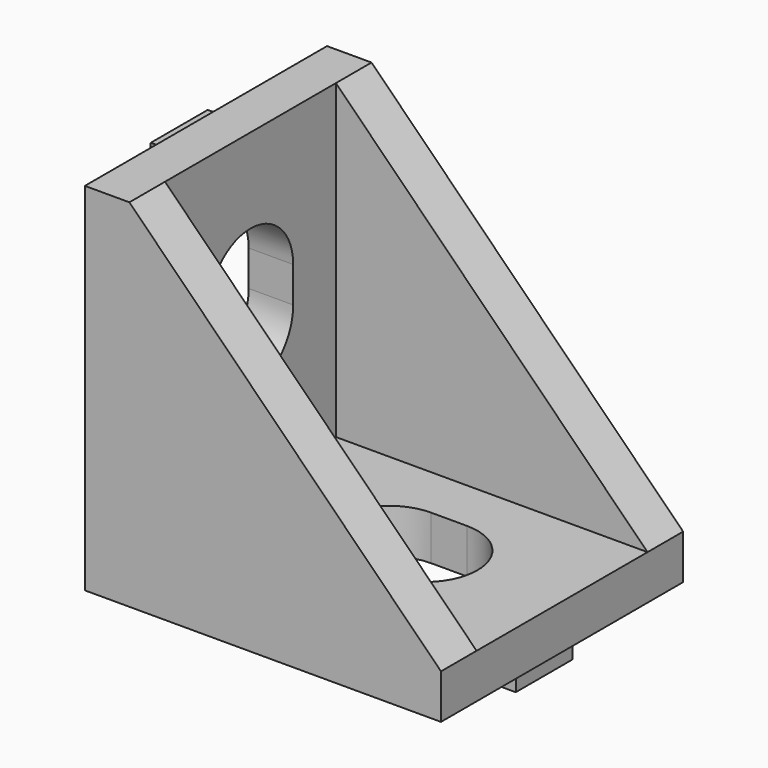
from build123d import *

# Parameters (mm, degrees)
F0_W     = 2.5
F0_H     = 8
F0_W_2   = 8
F0_H_2   = 2.5
F1_DEPTH = 17
F2_START = 2.5
F2_DEPTH = 12
F3_START = 5.5
F3_DEPTH = 6
F4_R     = 2.99999
F5_START = 6.5
F0_W_3   = 1.5
F0_H_3   = 1.5
F5_DEPTH = 4


# Not quite as in the source:
# - a fillet or chamfer is up to 0.001 mm smaller than in the source, because OpenCascade refuses the exact size


with BuildPart() as f1:
    # F0 (on Front) → F1 (new body)
    with BuildSketch(Plane.XZ):
        Polygon((20, 2.5), (2.5, 20), (2.5, 15.25), (2.5, 7.25), (2.5, 2.5), (7.25, 2.5), (15.25, 2.5), align=None)
        Polygon((20, 0), (20, 2.5), (15.25, 2.5), (15.25, 0), (16.5, 0), (19, 0), align=None)
        Polygon((2.5, 20), (0, 20), (0, 19), (0, 16.5), (0, 15.25), (2.5, 15.25), align=None)
        Polygon((2.5, 2.5), (2.5, 7.25), (0, 7.25), (0, 6), (0, 3.5), (0, 0), (3.5, 0), (6, 0), (7.25, 0), (7.25, 2.5), align=None)
        with Locations((1.25, 11.25)):
            Rectangle(F0_W, F0_H)
        with Locations((11.25, 1.25)):
            Rectangle(F0_W_2, F0_H_2)
    extrude(amount=F1_DEPTH)

    # F0 (on Front) → F2 (cut)
    with BuildSketch(Plane.XZ.offset(F2_START)):
        Polygon((20, 2.5), (2.5, 20), (2.5, 15.25), (2.5, 7.25), (2.5, 2.5), (7.25, 2.5), (15.25, 2.5), align=None)
    extrude(amount=F2_DEPTH, mode=Mode.SUBTRACT)

    # F0 (on Front) → F3 (cut)
    with BuildSketch(Plane.XZ.offset(F3_START)):
        with Locations((1.25, 11.25)):
            Rectangle(F0_W, F0_H)
        with Locations((11.25, 1.25)):
            Rectangle(F0_W_2, F0_H_2)
    extrude(amount=F3_DEPTH, mode=Mode.SUBTRACT)

    # F4 (radius 3 in the source; OpenCascade refuses exactly that, so slightly less here)
    f4_edges = [f1.edges().sort_by_distance(p)[0] for p in [
        (1.25, -11.5, 7.25),
        (1.25, -5.5, 7.25),
        (1.25, -11.5, 15.25),
        (1.25, -5.5, 15.25),
        (7.25, -11.5, 1.25),
        (7.25, -5.5, 1.25),
        (15.25, -11.5, 1.25),
        (15.25, -5.5, 1.25),
    ]]
    fillet(f4_edges, radius=F4_R)

    # F0 (on Front) → F5 (join)
    with BuildSketch(Plane.XZ.offset(F5_START)):
        with Locations((-0.75, 17.75)):
            Rectangle(F0_W_3, F0_H_2)
        with Locations((-0.75, 4.75)):
            Rectangle(F0_W_3, F0_H_2)
        with Locations((4.75, -0.75)):
            Rectangle(F0_W, F0_H_3)
        with Locations((17.75, -0.75)):
            Rectangle(F0_W, F0_H_3)
    extrude(amount=F5_DEPTH)


solid = f1.part
